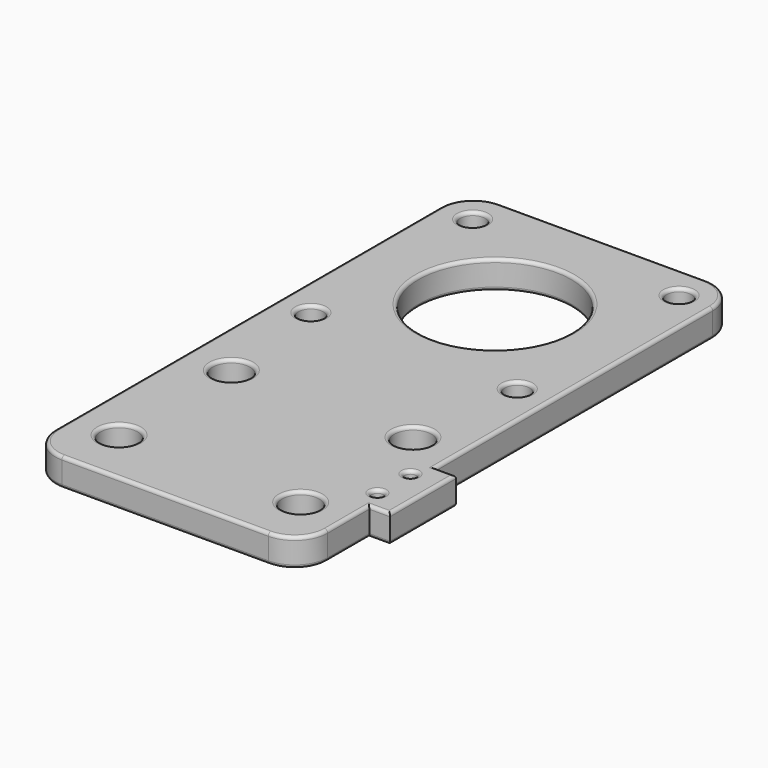
from build123d import *

# Parameters (mm, degrees)
F0_R     = 2.8575
F0_R_2   = 0.889
F0_R_3   = 1.905
F0_R_4   = 11.7475
F1_DEPTH = 4.318
F2_W     = 12.7
F2_H     = 4.318
F3_DEPTH = 3.175
F4_R     = 5.08
F5_R     = 0.508


# Not quite as in the source:
# - a feature names something its author has since deleted; it is built from what else it names


with BuildPart() as f1:
    # F0 (on Top) → F1 (new body)
    with BuildSketch(Plane.XY):
        Polygon((0, -20.7006), (0, 0), (0, 63.5), (-41.91, 63.5), (-41.91, 19), (-41.91, 0), (-41.91, -20.7006), align=None)
        with Locations((-34.925, -12.09)):
            Circle(F0_R, mode=Mode.SUBTRACT)
        with Locations((-34.925, 9.5)):
            Circle(F0_R, mode=Mode.SUBTRACT)
        with Locations((-6.985, -12.09)):
            Circle(F0_R, mode=Mode.SUBTRACT)
        with Locations((-1.27, -4.47)):
            Circle(F0_R_2, mode=Mode.SUBTRACT)
        with Locations((-6.985, 9.5)):
            Circle(F0_R, mode=Mode.SUBTRACT)
        with Locations((-1.27, 1.88)):
            Circle(F0_R_2, mode=Mode.SUBTRACT)
        with Locations((-36.83, 27.178)):
            Circle(F0_R_3, mode=Mode.SUBTRACT)
        with Locations((-36.83, 58.293)):
            Circle(F0_R_3, mode=Mode.SUBTRACT)
        with Locations((-5.08, 27.178)):
            Circle(F0_R_3, mode=Mode.SUBTRACT)
        with Locations((-20.955, 42.7355)):
            Circle(F0_R_4, mode=Mode.SUBTRACT)
        with Locations((-5.08, 58.293)):
            Circle(F0_R_3, mode=Mode.SUBTRACT)
    extrude(amount=F1_DEPTH)

    # F2 (on face) → F3 (join)
    with BuildSketch(Plane.YZ):
        with Locations((-1.2696, 2.159)):
            Rectangle(F2_W, F2_H)
    extrude(amount=F3_DEPTH)

    # F4
    f4_edges = [f1.edges().sort_by_distance(p)[0] for p in [
        (0, 63.5, 2.159),
        (-41.91, 63.5, 2.159),
        (0, -20.7006, 2.159),
        (-41.91, -20.7006, 2.159),
    ]]
    fillet(f4_edges, radius=F4_R)

    # F5
    f5_edges = [f1.edges().sort_by_distance(p)[0] for p in [
        (0, 31.7502, 4.318),
        (-37.7825, 9.5, 4.318),
        (-32.7025, 42.7355, 4.318),
        (0, 31.7502, 0),
        (-37.7825, 9.5, 0),
        (-37.7825, -12.09, 4.318),
        (-37.7825, -12.09, 0),
        (-32.7025, 42.7355, 0),
        (-1.487898, 62.012102, 4.318),
        (1.5875, 5.0804, 4.318),
        (-20.955, 63.5, 4.318),
        (3.175, -1.2696, 4.318),
        (-40.422102, 62.012102, 4.318),
        (1.5875, -7.6196, 4.318),
        (-41.91, 21.3997, 4.318),
        (0, -11.6201, 4.318),
        (-40.422102, -19.212702, 4.318),
        (-1.487898, -19.212702, 4.318),
        (-20.955, -20.7006, 4.318),
        (-9.8425, -12.09, 4.318),
        (-2.159, -4.47, 4.318),
        (-9.8425, 9.5, 4.318),
        (-2.159, 1.88, 4.318),
        (-38.735, 27.178, 4.318),
        (-38.735, 58.293, 4.318),
        (-6.985, 27.178, 4.318),
        (-6.985, 58.293, 4.318),
        (0, -11.6201, 0),
        (-1.487898, -19.212702, 0),
        (1.5875, -7.6196, 0),
        (-20.955, -20.7006, 0),
        (3.175, -1.2696, 0),
        (-40.422102, -19.212702, 0),
        (1.5875, 5.0804, 0),
        (-41.91, 21.3997, 0),
        (-40.422102, 62.012102, 0),
        (-1.487898, 62.012102, 0),
        (-20.955, 63.5, 0),
        (-9.8425, -12.09, 0),
        (-2.159, -4.47, 0),
        (-9.8425, 9.5, 0),
        (-2.159, 1.88, 0),
        (-38.735, 27.178, 0),
        (-38.735, 58.293, 0),
        (-6.985, 27.178, 0),
        (-6.985, 58.293, 0),
    ]]
    fillet(f5_edges, radius=F5_R)


solid = f1.part
